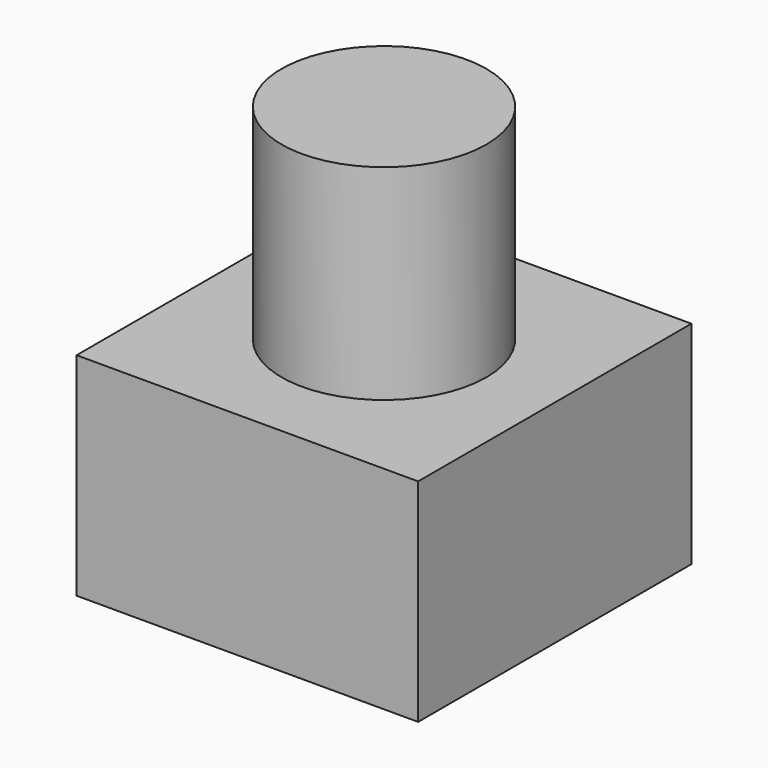
from build123d import *

# Parameters (mm, degrees)
F0_R     = 15
F1_DEPTH = 30
F2_W     = 50
F2_H     = 50
F3_DEPTH = 1
F4_W     = 50
F4_H     = 50
F4_W_2   = 30
F4_H_2   = 30
F5_DEPTH = 30


with BuildPart() as f1:
    # F0 (on Top) → F1 (new body)
    with BuildSketch(Plane.XY):
        Circle(F0_R)
    extrude(amount=F1_DEPTH)

    # F2 (on face) → F3 (join)
    with BuildSketch(Plane(origin=(0, 0, 0), x_dir=(1, 0, 0), z_dir=(0, 0, -1))):
        Rectangle(F2_W, F2_H)
        Polygon((15, 0), (15, -15), (0, -15), (-15, -15), (-15, 3.9e-09), (-15, 15), (0, 15), (15, 15), align=None, mode=Mode.SUBTRACT)
        with BuildLine():
            Line((0, -15), (15, -15))
            Line((15, -15), (15, 0))
            ThreePointArc((15, 0), (10.6066017178, -10.6066017178), (0, -15))
        make_face()
        with BuildLine():
            Line((-15, -15), (0, -15))
            ThreePointArc((0, -15), (-10.6066017192, -10.6066017164), (-15, 3.9e-09))
            Line((-15, 3.9e-09), (-15, -15))
        make_face()
        with BuildLine():
            ThreePointArc((-15, 3.9e-09), (-10.6066017192, -10.6066017164), (0, -15))
            ThreePointArc((0, -15), (10.6066017178, -10.6066017178), (15, 0))
            ThreePointArc((15, 0), (10.6066017178, 10.6066017178), (0, 15))
            ThreePointArc((0, 15), (-10.6066017164, 10.6066017192), (-15, 3.9e-09))
        make_face()
        with BuildLine():
            ThreePointArc((0, 15), (10.6066017178, 10.6066017178), (15, 0))
            Line((15, 0), (15, 15))
            Line((15, 15), (0, 15))
        make_face()
        with BuildLine():
            Line((-15, 15), (-15, 3.9e-09))
            ThreePointArc((-15, 3.9e-09), (-10.6066017164, 10.6066017192), (0, 15))
            Line((0, 15), (-15, 15))
        make_face()
    extrude(amount=F3_DEPTH)

    # F4 (on face) → F5 (join)
    with BuildSketch(Plane(origin=(0, 0, -1), x_dir=(1, 0, 0), z_dir=(0, 0, -1))):
        Rectangle(F4_W, F4_H)
        Rectangle(F4_W_2, F4_H_2, mode=Mode.SUBTRACT)
    extrude(amount=F5_DEPTH)


solid = f1.part
